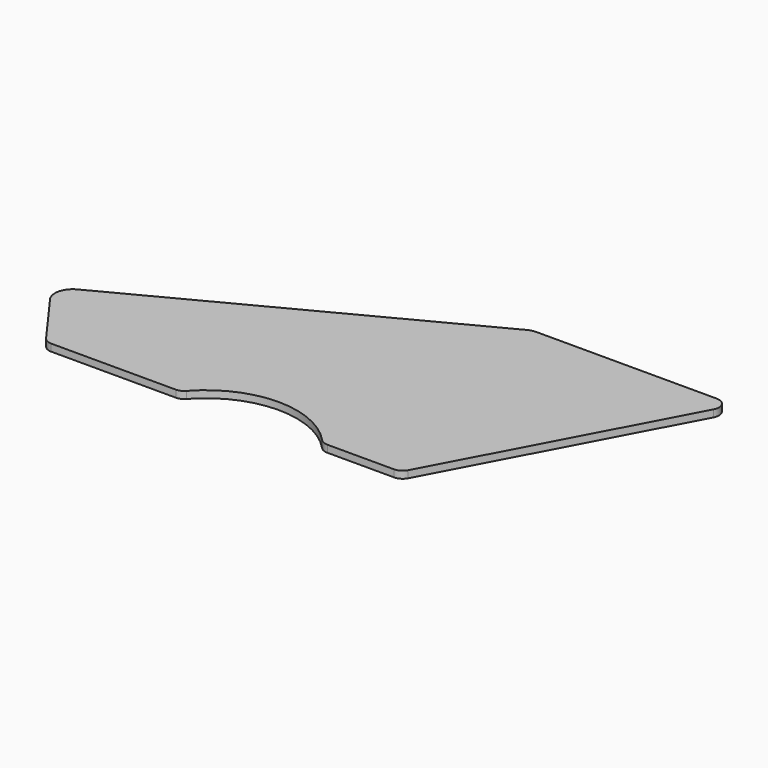
from build123d import *

# Parameters (mm, degrees)
F1_DEPTH = 2
F2_DEPTH = 1


# Not quite as in the source:
# - a feature names something its author has since deleted; it is built from what else it names


with BuildPart() as f1:
    # F0 (on Top) → F1 (new body)
    with BuildSketch(Plane.XY):
        with BuildLine():
            ThreePointArc((5.132071007, 2.6840715959), (2.5813003046, -0.6052114789), (3.40420502, -4.6854862431))
            Line((3.40420502, -4.6854862431), (14.383941925, -19.7977976106))
            ThreePointArc((14.383941925, -19.7977976106), (15.4490214089, -20.7074614263), (16.8109929081, -21.0344418537))
            Line((16.8109929081, -21.0344418537), (51.8963127054, -21.0344418537))
            ThreePointArc((51.8963127054, -21.0344418537), (53.12065768, -20.7732334455), (54.1317965199, -20.035094776))
            ThreePointArc((54.1317965199, -20.035094776), (73.0425506447, -11.4896803777), (92.0885582947, -19.7292387035))
            ThreePointArc((92.0885582947, -19.7292387035), (93.0892746148, -20.4413889466), (94.2915113407, -20.6928208003))
            Line((94.2915113407, -20.6928208003), (113.1330302084, -20.6928208003))
            ThreePointArc((113.1330302084, -20.6928208003), (114.6781444331, -20.2643227024), (115.781872987, -19.1012354886))
            Line((115.781872987, -19.1012354886), (150.1493414199, 45.5345719401))
            ThreePointArc((150.1493414199, 45.5345719401), (150.0720005434, 48.4881008532), (147.5004986413, 49.9429866284))
            Line((147.5004986413, 49.9429866284), (96.7218968968, 49.9429866284))
            ThreePointArc((96.7218968968, 49.9429866284), (95.5288247883, 49.7985585766), (94.4046779119, 49.373618206))
            Line((94.4046779119, 49.373618206), (5.132071007, 2.6840715959))
        make_face()
        with BuildLine():
            Line((83.7633376258, 38.1656639161), (96.7218969194, 44.9429865363))
            Line((96.7218969194, 44.9429865363), (144.1719395233, 44.9429865363))
            Line((144.1719395233, 44.9429865363), (141.3464313092, 39.6289784601))
            Line((141.3464313092, 39.6289784601), (137.1905609573, 31.8129231027))
            Line((137.1905609573, 31.8129231027), (111.931308915, -15.6928207082))
            Line((111.931308915, -15.6928207082), (103.8109142352, -15.6928207082))
            Line((103.8109142352, -15.6928207082), (95.14885507, -15.6928207082))
            ThreePointArc((95.14885507, -15.6928207082), (73.0119644332, -6.489765959), (51.0202089869, -16.0344417616))
            Line((51.0202089869, -16.0344417616), (18.1341059978, -16.0344417616))
            Line((18.1341059978, -16.0344417616), (17.830043854, -16.0344417616))
            Line((17.830043854, -16.0344417616), (14.9430452948, -12.0608291403))
            Line((14.9430452948, -12.0608291403), (7.4492901291, -1.7465600138))
            Line((7.4492901291, -1.7465600138), (45.2243497545, 18.0097848295))
            Line((45.2243497545, 18.0097848295), (49.4777560689, 20.234315055))
            Line((49.4777560689, 20.234315055), (79.3327060482, 35.8484449312))
            Line((79.3327060482, 35.8484449312), (83.7633376258, 38.1656639161))
        make_face(mode=Mode.SUBTRACT)
        Polygon((144.1719395233, 44.9429865363), (96.7218969194, 44.9429865363), (83.7633376258, 38.1656639161), (95.5301042855, 15.6670531815), (141.3464313092, 39.6289784601), align=None)
        Polygon((103.8606077396, -11.0500555872), (79.3327060482, 35.8484449312), (49.4777560689, 20.234315055), align=None)
        Polygon((58.1843801115, 10.554375987), (45.2243497545, 18.0097848295), (7.4492901291, -1.7465600138), (14.9430452948, -12.0608291403), align=None)
        Polygon((95.5301042855, 15.6670531815), (83.7633376258, 38.1656639161), (79.3327060482, 35.8484449312), (103.8606077396, -11.0500555872), (49.4777560689, 20.234315055), (45.2243497545, 18.0097848295), (58.1843801115, 10.554375987), (14.9430452948, -12.0608291403), (17.830043854, -16.0344417616), (18.1341059978, -16.0344417616), (63.3220791259, 7.5988546181), (103.8109142352, -15.6928207082), (111.931308915, -15.6928207082), (97.8473232704, 11.236421604), (137.1905609573, 31.8129231027), (141.3464313092, 39.6289784601), align=None)
        with BuildLine():
            Line((95.14885507, -15.6928207082), (103.8109142352, -15.6928207082))
            Line((103.8109142352, -15.6928207082), (63.3220791259, 7.5988546181))
            Line((63.3220791259, 7.5988546181), (18.1341059978, -16.0344417616))
            Line((18.1341059978, -16.0344417616), (51.0202089869, -16.0344417616))
            ThreePointArc((51.0202089869, -16.0344417616), (73.0119644332, -6.489765959), (95.14885507, -15.6928207082))
        make_face()
        Polygon((111.931308915, -15.6928207082), (137.1905609573, 31.8129231027), (97.8473232704, 11.236421604), align=None)
    extrude(amount=F1_DEPTH)

    # F0 (on Top) → F2 (cut)
    with BuildSketch(Plane.XY):
        Polygon((144.1719395233, 44.9429865363), (96.7218969194, 44.9429865363), (83.7633376258, 38.1656639161), (95.5301042855, 15.6670531815), (141.3464313092, 39.6289784601), align=None)
        Polygon((103.8606077396, -11.0500555872), (79.3327060482, 35.8484449312), (49.4777560689, 20.234315055), align=None)
        Polygon((111.931308915, -15.6928207082), (137.1905609573, 31.8129231027), (97.8473232704, 11.236421604), align=None)
        Polygon((58.1843801115, 10.554375987), (45.2243497545, 18.0097848295), (7.4492901291, -1.7465600138), (14.9430452948, -12.0608291403), align=None)
        with BuildLine():
            Line((95.14885507, -15.6928207082), (103.8109142352, -15.6928207082))
            Line((103.8109142352, -15.6928207082), (63.3220791259, 7.5988546181))
            Line((63.3220791259, 7.5988546181), (18.1341059978, -16.0344417616))
            Line((18.1341059978, -16.0344417616), (51.0202089869, -16.0344417616))
            ThreePointArc((51.0202089869, -16.0344417616), (73.0119644332, -6.489765959), (95.14885507, -15.6928207082))
        make_face()
    extrude(amount=F2_DEPTH, mode=Mode.SUBTRACT)


solid = f1.part
